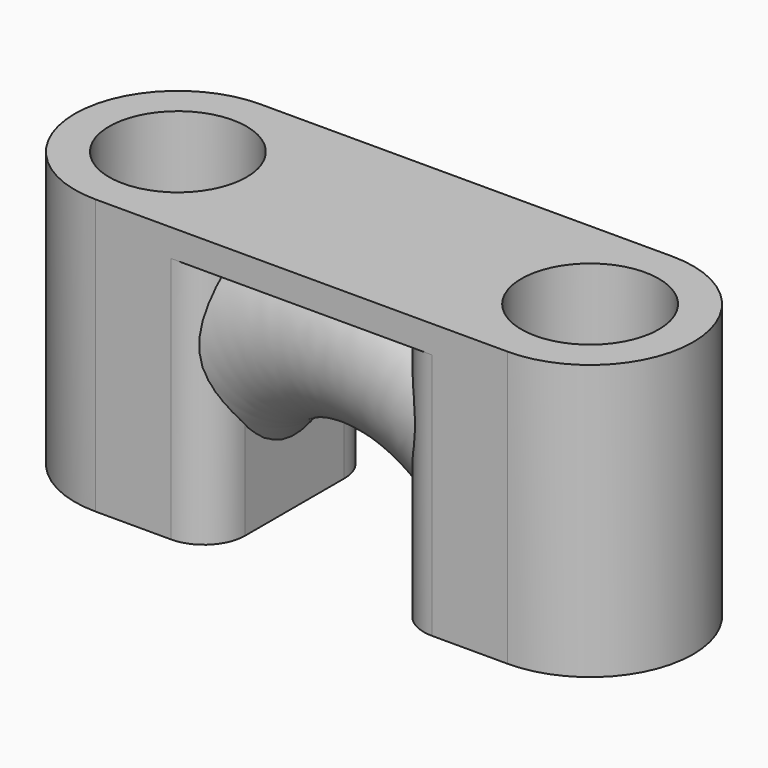
from build123d import *

# Parameters (mm, degrees)
F0_R     = 5
F1_DEPTH = 20
F3_ANGLE = 180
F4_W     = 13
F4_H     = 18
F5_DEPTH = 25
F6_R     = 3


with BuildPart() as f1:
    # F0 (on Top) → F1 (new body)
    with BuildSketch(Plane.XY):
        with BuildLine():
            ThreePointArc((-15, 7.5), (-9.6966991411, 5.3033008589), (-7.5, 0))
            ThreePointArc((-7.5, 0), (-9.6966991411, -5.3033008589), (-15, -7.5))
            Line((-15, -7.5), (0, -7.5))
            Line((0, -7.5), (5, -7.5))
            Line((5, -7.5), (15, -7.5))
            ThreePointArc((15, -7.5), (7.5, 0), (15, 7.5))
            Line((15, 7.5), (0, 7.5))
            Line((0, 7.5), (-15, 7.5))
        make_face()
        with BuildLine():
            ThreePointArc((-15, -7.5), (-9.6966991411, -5.3033008589), (-7.5, 0))
            ThreePointArc((-7.5, 0), (-9.6966991411, 5.3033008589), (-15, 7.5))
            ThreePointArc((-15, 7.5), (-22.5, 0), (-15, -7.5))
        make_face()
        with Locations((-15, 0)):
            Circle(F0_R, mode=Mode.SUBTRACT)
        with BuildLine():
            ThreePointArc((22.5, 0), (20.3033008589, 5.3033008589), (15, 7.5))
            ThreePointArc((15, 7.5), (7.5, 0), (15, -7.5))
            ThreePointArc((15, -7.5), (20.3033008589, -5.3033008589), (22.5, 0))
        make_face()
        with Locations((15, 0)):
            Circle(F0_R, mode=Mode.SUBTRACT)
    extrude(amount=F1_DEPTH)

    # F4 (on face) → F5 (cut)
    with BuildSketch(Plane.XZ.offset(7.5)):
        with Locations((0, 9)):
            Rectangle(F4_W, F4_H)
    extrude(amount=-F5_DEPTH, mode=Mode.SUBTRACT)

    # F6
    f6_edges = [f1.edges().sort_by_distance(p)[0] for p in [
        (-6.5, -7.5, 9),
        (-6.5, 7.5, 9),
        (6.5, 7.5, 9),
        (6.5, -7.5, 9),
    ]]
    fillet(f6_edges, radius=F6_R)


with BuildPart() as f3:
    # F2 (on Top) → F3 (revolve)
    with BuildSketch(Plane.XY):
        with BuildLine():
            Line((-17.5202840718, -4.3183524865), (-18.6972782109, -5.9505544354))
            ThreePointArc((-18.6972782109, -5.9505544354), (-7.9963954846, 0.1687840342), (-18.9796314418, 5.7655440199))
            Line((-18.9796314418, 5.7655440199), (-17.5202840718, 4.3183524865))
            ThreePointArc((-17.5202840718, 4.3183524865), (-10, 0), (-17.5202840718, -4.3183524865))
        make_face()
    revolve(axis=Axis((0, 4.9783602892, 0), (0, 1, 0)), revolution_arc=F3_ANGLE)


solid = Compound([f1.part, f3.part])
